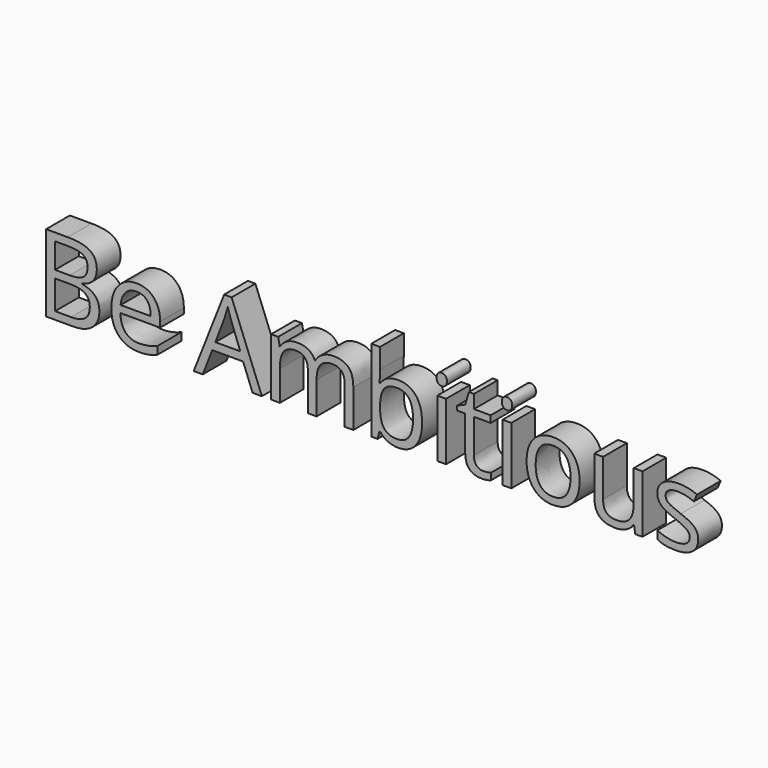
from build123d import *

# Parameters (mm, degrees)
F0_TEXT_SIZE = 90.6858075824
F1_DEPTH     = 25


# Not quite as in the source:
# - Text() gives the source's letters only with a copy of the font that has no kerning and outlines rounded to 1/6400 em; it was checked with that copy


with BuildPart() as f1:
    # F0 (on Front) → F1 (new body)
    with BuildSketch(Plane.XZ):
        with Locations((0, 0)):
            Text('Be Ambitious', F0_TEXT_SIZE, font='Open Sans', text_align=(TextAlign.LEFT, TextAlign.BOTTOM))
    extrude(amount=F1_DEPTH)


solid = f1.part
